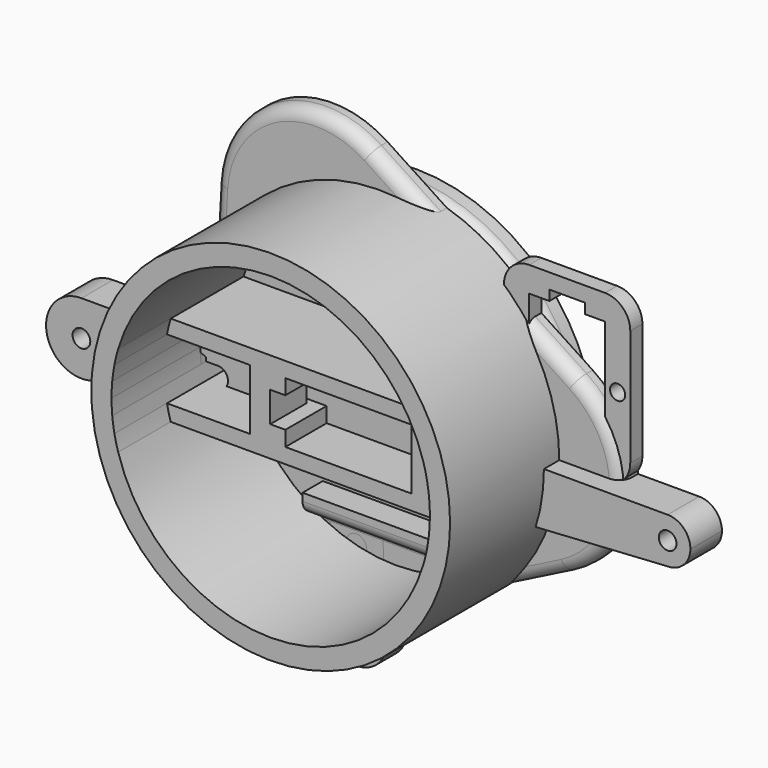
from build123d import *

# Parameters (mm, degrees)
F0_R          = 35.5
F0_W          = 29
F0_H          = 4
F0_R_2        = 1
F1_DEPTH      = 5
F2_DEPTH      = 5
F0_R_3        = 1.75
F3_DEPTH      = 3
F4_R          = 1.5
F5_DEPTH      = 3
F7_R          = 2.49999
F8_R          = 2.49999
F9_R          = 2.5
F11_DEPTH     = 31
F10_W         = 4
F10_H         = 3
F10_W_2       = 3
F12_DEPTH     = 18
F13_DEPTH     = 9
F14_DEPTH     = 9
F15_T4_DEPTH  = 14.302926823
F15_S5_R      = 31.5
F15_T6_DEPTH  = 9
F15_S7_R      = 35.5
F15_T8_DEPTH  = 9
F15_T12_DEPTH = 14.302926823
F15_S13_R     = 31.5
F15_T14_DEPTH = 9
F15_S15_R     = 35.5
F15_T16_DEPTH = 9
F17_DEPTH     = 4
F18_R         = 2.5
F6_R          = 2
F19_DEPTH     = 5
F20_DEPTH     = 3
F21_R         = 1.75
F22_DEPTH     = 7.8
F23_R         = 15
F24_DEPTH     = 2
F25_DEPTH     = 8


# Not quite as in the source:
# - a fillet or chamfer that OpenCascade refuses, or shapes differently, is made with other operations: its cross-section is extruded or revolved along the edge and cut away or added
# - a fillet or chamfer is up to 0.001 mm smaller than in the source, because OpenCascade refuses the exact size


with BuildPart() as f1:
    # F0 (on Front) → F1 (new body)
    with BuildSketch(Plane.XZ):
        Circle(F0_R)
        with Locations((0, -23.522429496)):
            Rectangle(F0_W, F0_H, mode=Mode.SUBTRACT)
        Polygon((-17.0606780064, 2.7416863016), (-13.6559690168, 3.1554426533), (-11.5952910104, 0.4137563518), (-12.9393219936, -2.7416863016), (-16.3440309832, -3.1554426533), (-18.4047089896, -0.4137563518), align=None, mode=Mode.SUBTRACT)
        Circle(F0_R_2, mode=Mode.SUBTRACT)
        Polygon((13.9117840481, 3.1093030377), (17.1486274427, 2.497074178), (18.2368433946, -0.6122288597), (16.0882159519, -3.1093030377), (12.8513725573, -2.497074178), (11.7631566054, 0.6122288597), align=None, mode=Mode.SUBTRACT)
        with Locations((0, 22.477570504)):
            Rectangle(F0_W, F0_H, mode=Mode.SUBTRACT)
        with Locations((0, 22.477570504)):
            Rectangle(F0_W, F0_H)
        with Locations((0, -23.522429496)):
            Rectangle(F0_W, F0_H)
    extrude(amount=-F1_DEPTH)

    # F0 (on Front) → F2 (join)
    with BuildSketch(Plane.XZ):
        with Locations((0, 22.477570504)):
            Rectangle(F0_W, F0_H)
        with Locations((0, -23.522429496)):
            Rectangle(F0_W, F0_H)
    extrude(amount=F2_DEPTH)

    # F0 (on Front) → F3 (join)
    with BuildSketch(Plane.XZ):
        Polygon((18.2368433946, -0.6122288597), (17.1486274427, 2.497074178), (13.9117840481, 3.1093030377), (11.7631566054, 0.6122288597), (12.8513725573, -2.497074178), (16.0882159519, -3.1093030377), align=None)
        with Locations((15, 0)):
            Circle(F0_R_3, mode=Mode.SUBTRACT)
        Polygon((-11.5952910104, 0.4137563518), (-13.6559690168, 3.1554426533), (-17.0606780064, 2.7416863016), (-18.4047089896, -0.4137563518), (-16.3440309832, -3.1554426533), (-12.9393219936, -2.7416863016), align=None)
        with Locations((-15, 0)):
            Circle(F0_R_3, mode=Mode.SUBTRACT)
    extrude(amount=-F3_DEPTH)

    # F7 (radius 2.5 in the source; OpenCascade refuses exactly that, so slightly less here)
    f7_edges = [f1.edges().sort_by_distance(p)[0] for p in [
        (0, -5, -25.522429),
        (0, 0, -25.522429),
    ]]
    fillet(f7_edges, radius=F7_R)

    # F8 (radius 2.5 in the source; OpenCascade refuses exactly that, so slightly less here)
    f8_edges = [f1.edges().sort_by_distance(p)[0] for p in [
        (0, -5, 24.477571),
        (0, 0, 24.477571),
    ]]
    fillet(f8_edges, radius=F8_R)

    # F9
    f9_edges = [f1.edges().sort_by_distance(p)[0] for p in [
        (-35.5, 0, 0),
    ]]
    fillet(f9_edges, radius=F9_R)


with BuildPart() as f5:
    # F4 (on Front) → F5 (new body)
    with BuildSketch(Plane.XZ):
        with BuildLine():
            Line((43.7464710474, 31.4150267243), (28.7464710474, 31.4150267243))
            ThreePointArc((28.7464710474, 31.4150267243), (25.2109371415, 29.9505606303), (23.7464710474, 26.4150267243))
            Line((23.7464710474, 26.4150267243), (23.7464710474, 3.4150267243))
            ThreePointArc((23.7464710474, 3.4150267243), (25.2109371415, -0.1205071816), (28.7464710474, -1.5849732757))
            Line((28.7464710474, -1.5849732757), (43.7464710474, -1.5849732757))
            ThreePointArc((43.7464710474, -1.5849732757), (47.2820049533, -0.1205071816), (48.7464710474, 3.4150267243))
            Line((48.7464710474, 3.4150267243), (48.7464710474, 26.4150267243))
            ThreePointArc((48.7464710474, 26.4150267243), (47.2820049533, 29.9505606303), (43.7464710474, 31.4150267243))
        make_face()
        with Locations((26.2464710474, 14.9150267243)):
            Circle(F4_R, mode=Mode.SUBTRACT)
        Polygon((28.7464710474, 3.4150267243), (28.7464710474, 26.4150267243), (32.7464710474, 26.4150267243), (32.7464710474, 28.4150267243), (39.7464710474, 28.4150267243), (39.7464710474, 26.4150267243), (43.7464710474, 26.4150267243), (43.7464710474, 3.4150267243), align=None, mode=Mode.SUBTRACT)
        with Locations((46.2464710474, 14.9150267243)):
            Circle(F4_R, mode=Mode.SUBTRACT)
    extrude(amount=F5_DEPTH)


with BuildPart() as f11:
    # F10 (on Front) → F11 (new body)
    with BuildSketch(Plane.XZ):
        with BuildLine():
            ThreePointArc((-31.5, 0), (-31.4641839985, 1.5017074653), (-31.3568174406, 3))
            Line((-31.3568174406, 3), (-35.3730123116, 3))
            ThreePointArc((-35.3730123116, 3), (-35.5, 0), (-35.3730123116, -3))
            Line((-35.3730123116, -3), (-31.3568174406, -3))
            ThreePointArc((-31.3568174406, -3), (-31.4641839985, -1.5017074653), (-31.5, 0))
        make_face()
        with BuildLine():
            ThreePointArc((30.9232921921, 6), (31.3554915769, 3.0138261353), (31.5, 0))
            ThreePointArc((31.5, 0), (31.3554915769, -3.0138261353), (30.9232921921, -6))
            ThreePointArc((30.9232921921, -6), (30.5919015125, -7.5090320181), (30.1869176962, -9))
            ThreePointArc((30.1869176962, -9), (0, -31.5), (-30.1869176962, -9))
            ThreePointArc((-30.1869176962, -9), (-30.5919015125, -7.5090320181), (-30.9232921921, -6))
            ThreePointArc((-30.9232921921, -6), (-31.1761609882, -4.5052176457), (-31.3568174406, -3))
            Line((-31.3568174406, -3), (-35.3730123116, -3))
            ThreePointArc((-35.3730123116, -3), (1.5013432213, -35.4682388699), (35.5, 0))
            ThreePointArc((35.5, 0), (1.5013432213, 35.4682388699), (-35.3730123116, 3))
            Line((-35.3730123116, 3), (-31.3568174406, 3))
            ThreePointArc((-31.3568174406, 3), (-31.1761609882, 4.5052176457), (-30.9232921921, 6))
            ThreePointArc((-30.9232921921, 6), (-30.5919015125, 7.5090320181), (-30.1869176962, 9))
            ThreePointArc((-30.1869176962, 9), (0, 31.5), (30.1869176962, 9))
            ThreePointArc((30.1869176962, 9), (30.5919015125, 7.5090320181), (30.9232921921, 6))
        make_face()
    extrude(amount=F11_DEPTH)

    # F10 (on Front) → F12 (join)
    with BuildSketch(Plane.XZ):
        with BuildLine():
            Line((22.5, 6), (30.9232921921, 6))
            ThreePointArc((30.9232921921, 6), (30.5919015125, 7.5090320181), (30.1869176962, 9))
            Line((30.1869176962, 9), (-30.1869176962, 9))
            ThreePointArc((-30.1869176962, 9), (-30.5919015125, 7.5090320181), (-30.9232921921, 6))
            Line((-30.9232921921, 6), (-14.5, 6))
            Line((-14.5, 6), (-10.5, 6))
            Line((-10.5, 6), (-7.5, 6))
            Line((-7.5, 6), (17.5, 6))
            Line((17.5, 6), (22.5, 6))
        make_face()
        with BuildLine():
            ThreePointArc((30.1869176962, -9), (30.5919015125, -7.5090320181), (30.9232921921, -6))
            Line((30.9232921921, -6), (22.5, -6))
            Line((22.5, -6), (17.5, -6))
            Line((17.5, -6), (-7.5, -6))
            Line((-7.5, -6), (-10.5, -6))
            Line((-10.5, -6), (-14.5, -6))
            Line((-14.5, -6), (-30.9232921921, -6))
            ThreePointArc((-30.9232921921, -6), (-30.5919015125, -7.5090320181), (-30.1869176962, -9))
            Line((-30.1869176962, -9), (30.1869176962, -9))
        make_face()
        Polygon((22.5, -6), (22.5, 0), (22.5, 6), (17.5, 6), (17.5, -6), align=None)
        Polygon((-10.5, 3), (-14.5, 3), (-14.5, 0), (-14.5, -3), (-10.5, -3), align=None)
        with Locations((-12.5, 4.5)):
            Rectangle(F10_W, F10_H)
        with Locations((-9, 4.5)):
            Rectangle(F10_W_2, F10_H)
        with Locations((-9, -4.5)):
            Rectangle(F10_W_2, F10_H)
        with Locations((-12.5, -4.5)):
            Rectangle(F10_W, F10_H)
    extrude(amount=F12_DEPTH)

    # F10 (on Front) → F13 (cut)
    with BuildSketch(Plane.XZ):
        Polygon((-10.5, 3), (-14.5, 3), (-14.5, 0), (-14.5, -3), (-10.5, -3), align=None)
    extrude(amount=F13_DEPTH, mode=Mode.SUBTRACT)

    # F10 (on Front) → F14 (cut)
    with BuildSketch(Plane.XZ):
        with BuildLine():
            ThreePointArc((-31.5, 0), (-31.4641839985, 1.5017074653), (-31.3568174406, 3))
            Line((-31.3568174406, 3), (-35.3730123116, 3))
            ThreePointArc((-35.3730123116, 3), (-35.5, 0), (-35.3730123116, -3))
            Line((-35.3730123116, -3), (-31.3568174406, -3))
            ThreePointArc((-31.3568174406, -3), (-31.4641839985, -1.5017074653), (-31.5, 0))
        make_face()
    extrude(amount=F14_DEPTH, mode=Mode.SUBTRACT)

    # F15: chamfer of 2 on 2 edges, made by hand


with BuildPart() as f15_tool2:
    # F15_s3 → F15_t4 (new body)
    with BuildSketch(Plane.YZ.offset(-26.2134514646)):
        Polygon((-9, 1), (-7, 3), (-9, 3), align=None)
    extrude(amount=-F15_T4_DEPTH)

    # F15_s5 → F15_t6 (cut, symmetric)
    with BuildSketch(Plane.XZ.offset(8)):
        Circle(F15_S5_R)
    extrude(amount=F15_T6_DEPTH, both=True, mode=Mode.SUBTRACT)

    # F15_s7 → F15_t8 (intersect, symmetric)
    with BuildSketch(Plane.XZ.offset(8)):
        Circle(F15_S7_R)
    extrude(amount=F15_T8_DEPTH, both=True, mode=Mode.INTERSECT)


with BuildPart() as f11_1:
    add(f11.part)

    # F15_t1: union F15_tool2
    add(f15_tool2.part)


with BuildPart() as f15_tool10:
    # F15_s11 → F15_t12 (new body)
    with BuildSketch(Plane.YZ.offset(-40.5163782876)):
        Polygon((-7, -3), (-9, -1), (-9, -3), align=None)
    extrude(amount=F15_T12_DEPTH)

    # F15_s13 → F15_t14 (cut, symmetric)
    with BuildSketch(Plane.XZ.offset(8)):
        Circle(F15_S13_R)
    extrude(amount=F15_T14_DEPTH, both=True, mode=Mode.SUBTRACT)

    # F15_s15 → F15_t16 (intersect, symmetric)
    with BuildSketch(Plane.XZ.offset(8)):
        Circle(F15_S15_R)
    extrude(amount=F15_T16_DEPTH, both=True, mode=Mode.INTERSECT)


with BuildPart() as f11_2:
    add(f11_1.part)

    # F15_t9: union F15_tool10
    add(f15_tool10.part)

    # F16 (on face) → F17 (join)
    with BuildSketch(Plane.XZ):
        with BuildLine():
            ThreePointArc((-33.3783015345, 12.0887959148), (-16.0094790364, 31.6851160797), (10.0699705918, 34.0418226933))
            Line((10.0699705918, 34.0418226933), (-1.6776871675, 41.7275132948))
            ThreePointArc((-1.6776871675, 41.7275132948), (-21.6466195422, 42.8418470936), (-32.5961271076, 26.1054112701))
            Line((-32.5961271076, 26.1054112701), (-33.3783015345, 12.0887959148))
        make_face()
        with BuildLine():
            Line((38.90601289, 15.1763685051), (27.1583551307, 22.8620591067))
            ThreePointArc((27.1583551307, 22.8620591067), (33.3494498241, 12.1681632316), (35.5, 0))
            ThreePointArc((35.5, 0), (32.6196756356, -14.0073823904), (24.4460979476, -25.7417616945))
            Line((24.4460979476, -25.7417616945), (36.9759301338, -19.4108369407))
            ThreePointArc((36.9759301338, -19.4108369407), (47.9254376992, -2.6744011172), (38.90601289, 15.1763685051))
        make_face()
        with BuildLine():
            Line((-6.3098857823, -41.2817797753), (6.2199464039, -34.9508550215))
            ThreePointArc((6.2199464039, -34.9508550215), (-19.4353759286, -29.7071735867), (-34.5160685394, -8.3000609988))
            Line((-34.5160685394, -8.3000609988), (-35.2982429663, -22.3166763541))
            ThreePointArc((-35.2982429663, -22.3166763541), (-26.278818157, -40.1674459764), (-6.3098857823, -41.2817797753))
        make_face()
    extrude(amount=F17_DEPTH)

    # F18
    f18_edges = [f11_2.edges().sort_by_distance(p)[0] for p in [
        (47.925438, -4, -2.674401),
        (-26.278818, -4, -40.167446),
        (-21.64662, -4, 42.841847),
        (-34.907156, -4, -15.308369),
        (-0.04497, -4, -38.116317),
        (30.711014, -4, -22.576299),
        (33.032184, -4, 19.019214),
        (4.196142, -4, 37.884668),
        (-32.987214, -4, 19.097104),
    ]]
    fillet(f18_edges, radius=F18_R)


with BuildPart() as f19:
    # F6 (on Front) → F19 (new body)
    with BuildSketch(Plane.XZ):
        with BuildLine():
            Line((-13.8065919992, -45.0317585825), (-13.8285924066, -45.5451014222))
            ThreePointArc((-13.8285924066, -45.5451014222), (-7.8285924066, -51.5451014222), (-1.8285924066, -45.5451014222))
            Line((-1.8285924066, -45.5451014222), (-1.850592814, -45.0317585825))
            ThreePointArc((-1.850592814, -45.0317585825), (-2.7682693631, -42.3212635392), (-4.8370166993, -40.3440943285))
            Line((-4.8370166993, -40.3440943285), (-4.346375486, -45.1927304275))
            ThreePointArc((-4.346375486, -45.1927304275), (-4.3330410036, -45.3686917032), (-4.3285924066, -45.5451014222))
            ThreePointArc((-4.3285924066, -45.5451014222), (-7.8285924066, -49.0451014222), (-11.3285924066, -45.5451014222))
            ThreePointArc((-11.3285924066, -45.5451014222), (-11.3112225723, -45.1968384056), (-11.2592854759, -44.8520321152))
            Line((-11.2592854759, -44.8520321152), (-10.807781171, -40.3369890668))
            ThreePointArc((-10.807781171, -40.3369890668), (-12.8850754746, -42.3152439976), (-13.8065919992, -45.0317585825))
        make_face()
        with BuildLine():
            Line((-12.3285924066, -10.5451014222), (-13.8065919992, -45.0317585825))
            ThreePointArc((-13.8065919992, -45.0317585825), (-12.8850754746, -42.3152439976), (-10.807781171, -40.3369890668))
            Line((-10.807781171, -40.3369890668), (-10.0952782738, -33.2119600947))
            ThreePointArc((-10.0952782738, -33.2119600947), (-11.2414756107, -31.3211350781), (-11.0255877564, -29.1205942327))
            Line((-11.0255877564, -29.1205942327), (-10.3881177664, -14.2462944639))
            ThreePointArc((-10.3881177664, -14.2462944639), (-11.8140575061, -12.634615227), (-12.3285924066, -10.5451014222))
        make_face()
        with BuildLine():
            ThreePointArc((-4.8370166993, -40.3440943285), (-2.7682693631, -42.3212635392), (-1.850592814, -45.0317585825))
            Line((-1.850592814, -45.0317585825), (-3.3285924066, -10.5451014222))
            ThreePointArc((-3.3285924066, -10.5451014222), (-3.8431273071, -12.634615227), (-5.2690670468, -14.2462944639))
            Line((-5.2690670468, -14.2462944639), (-4.6315970567, -29.1205942327))
            ThreePointArc((-4.6315970567, -29.1205942327), (-4.4051815545, -29.8169131651), (-4.3285924066, -30.5451014222))
            ThreePointArc((-4.3285924066, -30.5451014222), (-4.6510429476, -32.01247303), (-5.5589806554, -33.2094704842))
            Line((-5.5589806554, -33.2094704842), (-4.8370166993, -40.3440943285))
        make_face()
        with BuildLine():
            Line((-10.0952782738, -33.2119600947), (-10.807781171, -40.3369890668))
            ThreePointArc((-10.807781171, -40.3369890668), (-7.8214523594, -39.5451056705), (-4.8370166993, -40.3440943285))
            Line((-4.8370166993, -40.3440943285), (-5.5589806554, -33.2094704842))
            ThreePointArc((-5.5589806554, -33.2094704842), (-7.8266715372, -34.045100895), (-10.0952782738, -33.2119600947))
        make_face()
        with BuildLine():
            ThreePointArc((-4.8370166993, -40.3440943285), (-7.8214523594, -39.5451056705), (-10.807781171, -40.3369890668))
            Line((-10.807781171, -40.3369890668), (-11.2592854759, -44.8520321152))
            ThreePointArc((-11.2592854759, -44.8520321152), (-7.656306273, -42.0493443528), (-4.346375486, -45.1927304275))
            Line((-4.346375486, -45.1927304275), (-4.8370166993, -40.3440943285))
        make_face()
        with BuildLine():
            ThreePointArc((-3.3285924066, -10.5451014222), (-7.8285924066, -6.0451014222), (-12.3285924066, -10.5451014222))
            ThreePointArc((-12.3285924066, -10.5451014222), (-11.8140575061, -12.634615227), (-10.3881177664, -14.2462944639))
            ThreePointArc((-10.3881177664, -14.2462944639), (-7.8285924066, -15.0451014222), (-5.2690670468, -14.2462944639))
            ThreePointArc((-5.2690670468, -14.2462944639), (-3.8431273071, -12.634615227), (-3.3285924066, -10.5451014222))
        make_face()
        with Locations((-7.8285924066, -10.5451014222)):
            Circle(F6_R, mode=Mode.SUBTRACT)
        with BuildLine():
            ThreePointArc((-11.0255877564, -29.1205942327), (-11.2414756107, -31.3211350781), (-10.0952782738, -33.2119600947))
            Line((-10.0952782738, -33.2119600947), (-9.8285924066, -30.5451014222))
            ThreePointArc((-9.8285924066, -30.5451014222), (-7.8285924066, -28.5451014222), (-5.8285924066, -30.5451014222))
            Line((-5.8285924066, -30.5451014222), (-5.5589806554, -33.2094704842))
            ThreePointArc((-5.5589806554, -33.2094704842), (-4.6510429476, -32.01247303), (-4.3285924066, -30.5451014222))
            ThreePointArc((-4.3285924066, -30.5451014222), (-4.4051815545, -29.8169131651), (-4.6315970567, -29.1205942327))
            ThreePointArc((-4.6315970567, -29.1205942327), (-7.8285924066, -27.0451014222), (-11.0255877564, -29.1205942327))
        make_face()
        with BuildLine():
            Line((-9.8285924066, -30.5451014222), (-10.0952782738, -33.2119600947))
            ThreePointArc((-10.0952782738, -33.2119600947), (-7.8266715372, -34.045100895), (-5.5589806554, -33.2094704842))
            Line((-5.5589806554, -33.2094704842), (-5.8285924066, -30.5451014222))
            ThreePointArc((-5.8285924066, -30.5451014222), (-7.8285924066, -32.5451014222), (-9.8285924066, -30.5451014222))
        make_face()
        with BuildLine():
            ThreePointArc((-4.346375486, -45.1927304275), (-7.656306273, -42.0493443528), (-11.2592854759, -44.8520321152))
            Line((-11.2592854759, -44.8520321152), (-11.3285924066, -45.5451014222))
            ThreePointArc((-11.3285924066, -45.5451014222), (-7.8285924066, -49.0451014222), (-4.3285924066, -45.5451014222))
            ThreePointArc((-4.3285924066, -45.5451014222), (-4.3330410036, -45.3686917032), (-4.346375486, -45.1927304275))
        make_face()
        with Locations((-7.8285924066, -45.5451014222)):
            Circle(F6_R, mode=Mode.SUBTRACT)
        with BuildLine():
            ThreePointArc((-5.2690670468, -14.2462944639), (-7.8285924066, -15.0451014222), (-10.3881177664, -14.2462944639))
            Line((-10.3881177664, -14.2462944639), (-11.0255877564, -29.1205942327))
            ThreePointArc((-11.0255877564, -29.1205942327), (-7.8285924066, -27.0451014222), (-4.6315970567, -29.1205942327))
            Line((-4.6315970567, -29.1205942327), (-5.2690670468, -14.2462944639))
        make_face()
        with BuildLine():
            ThreePointArc((-5.8285924066, -30.5451014222), (-7.8285924066, -28.5451014222), (-9.8285924066, -30.5451014222))
            ThreePointArc((-9.8285924066, -30.5451014222), (-7.8285924066, -32.5451014222), (-5.8285924066, -30.5451014222))
        make_face()
    extrude(amount=-F19_DEPTH)

    # F6 (on Front) → F20 (cut)
    with BuildSketch(Plane.XZ):
        with BuildLine():
            Line((-10.0952782738, -33.2119600947), (-10.807781171, -40.3369890668))
            ThreePointArc((-10.807781171, -40.3369890668), (-7.8214523594, -39.5451056705), (-4.8370166993, -40.3440943285))
            Line((-4.8370166993, -40.3440943285), (-5.5589806554, -33.2094704842))
            ThreePointArc((-5.5589806554, -33.2094704842), (-7.8266715372, -34.045100895), (-10.0952782738, -33.2119600947))
        make_face()
        with BuildLine():
            ThreePointArc((-4.8370166993, -40.3440943285), (-7.8214523594, -39.5451056705), (-10.807781171, -40.3369890668))
            Line((-10.807781171, -40.3369890668), (-11.2592854759, -44.8520321152))
            ThreePointArc((-11.2592854759, -44.8520321152), (-7.656306273, -42.0493443528), (-4.346375486, -45.1927304275))
            Line((-4.346375486, -45.1927304275), (-4.8370166993, -40.3440943285))
        make_face()
        with BuildLine():
            ThreePointArc((-4.346375486, -45.1927304275), (-7.656306273, -42.0493443528), (-11.2592854759, -44.8520321152))
            Line((-11.2592854759, -44.8520321152), (-11.3285924066, -45.5451014222))
            ThreePointArc((-11.3285924066, -45.5451014222), (-7.8285924066, -49.0451014222), (-4.3285924066, -45.5451014222))
            ThreePointArc((-4.3285924066, -45.5451014222), (-4.3330410036, -45.3686917032), (-4.346375486, -45.1927304275))
        make_face()
        with Locations((-7.8285924066, -45.5451014222)):
            Circle(F6_R, mode=Mode.SUBTRACT)
        with BuildLine():
            Line((-9.8285924066, -30.5451014222), (-10.0952782738, -33.2119600947))
            ThreePointArc((-10.0952782738, -33.2119600947), (-7.8266715372, -34.045100895), (-5.5589806554, -33.2094704842))
            Line((-5.5589806554, -33.2094704842), (-5.8285924066, -30.5451014222))
            ThreePointArc((-5.8285924066, -30.5451014222), (-7.8285924066, -32.5451014222), (-9.8285924066, -30.5451014222))
        make_face()
        with BuildLine():
            ThreePointArc((-5.8285924066, -30.5451014222), (-7.8285924066, -28.5451014222), (-9.8285924066, -30.5451014222))
            ThreePointArc((-9.8285924066, -30.5451014222), (-7.8285924066, -32.5451014222), (-5.8285924066, -30.5451014222))
        make_face()
    extrude(amount=-F20_DEPTH, mode=Mode.SUBTRACT)


with BuildPart() as f22:
    # F21 (on Front) → F22 (new body)
    with BuildSketch(Plane.XZ):
        with BuildLine():
            Line((59.9833536744, 0), (-56.0166463256, 0))
            ThreePointArc((-56.0166463256, 0), (-52.2996435239, -1.0683990212), (-49.7172813379, -3.9474599509))
            ThreePointArc((-49.7172813379, -3.9474599509), (-48.9900218702, -3.2528480177), (-48.0166463256, -3))
            Line((-48.0166463256, -3), (-29.0166463256, -3))
            ThreePointArc((-29.0166463256, -3), (-28.0341015748, -3.2579879987), (-27.3050415779, -3.9653941874))
            ThreePointArc((-27.3050415779, -3.9653941874), (-19.4385197238, -0.2198002349), (-14.0162597141, -7.039678278))
            ThreePointArc((-14.0162597141, -7.039678278), (-15.7686933898, -11.6725011402), (-20.1485590491, -13.9856912031))
            Line((-20.1485590491, -13.9856912031), (59.9833536744, -9))
            ThreePointArc((59.9833536744, -9), (55.4833536744, -4.5), (59.9833536744, 0))
        make_face()
        with BuildLine():
            ThreePointArc((-49.0166463256, -7), (-49.2551655416, -8.8117333157), (-49.9544684991, -10.5))
            Line((-49.9544684991, -10.5), (-27.1011733191, -10.5))
            ThreePointArc((-27.1011733191, -10.5), (-27.8218206103, -8.6780741057), (-28.0093082494, -6.7277933905))
            ThreePointArc((-28.0093082494, -6.7277933905), (-28.494912093, -6.9307494375), (-29.0166463256, -7))
            Line((-29.0166463256, -7), (-48.0166463256, -7))
            ThreePointArc((-48.0166463256, -7), (-48.537212712, -6.9310646383), (-49.0218936662, -6.7290106374))
            ThreePointArc((-49.0218936662, -6.7290106374), (-49.0179582837, -6.8644799192), (-49.0166463256, -7))
        make_face()
        with BuildLine():
            ThreePointArc((-49.7172813379, -3.9474599509), (-52.2996435239, -1.0683990212), (-56.0166463256, 0))
            ThreePointArc((-56.0166463256, 0), (-62.0788241521, -10.5), (-49.9544684991, -10.5))
            ThreePointArc((-49.9544684991, -10.5), (-49.2551655416, -8.8117333157), (-49.0166463256, -7))
            ThreePointArc((-49.0166463256, -7), (-49.0179582837, -6.8644799192), (-49.0218936662, -6.7290106374))
            ThreePointArc((-49.0218936662, -6.7290106374), (-49.9569313259, -5.4850712501), (-49.7172813379, -3.9474599509))
        make_face()
        with Locations((-56.0166463256, -7)):
            Circle(F21_R, mode=Mode.SUBTRACT)
        with BuildLine():
            Line((-29.0166463256, -3), (-48.0166463256, -3))
            ThreePointArc((-48.0166463256, -3), (-46.6024327632, -3.5857864376), (-46.0166463256, -5))
            ThreePointArc((-46.0166463256, -5), (-46.6024327632, -6.4142135624), (-48.0166463256, -7))
            Line((-48.0166463256, -7), (-29.0166463256, -7))
            ThreePointArc((-29.0166463256, -7), (-31.0166463256, -5), (-29.0166463256, -3))
        make_face()
        with BuildLine():
            ThreePointArc((-29.0166463256, -7), (-28.494912093, -6.9307494375), (-28.0093082494, -6.7277933905))
            ThreePointArc((-28.0093082494, -6.7277933905), (-27.7992875798, -5.3103625251), (-27.3050415779, -3.9653941874))
            ThreePointArc((-27.3050415779, -3.9653941874), (-28.0341015748, -3.2579879987), (-29.0166463256, -3))
            ThreePointArc((-29.0166463256, -3), (-31.0166463256, -5), (-29.0166463256, -7))
        make_face()
        with BuildLine():
            ThreePointArc((-48.0166463256, -3), (-48.9900218702, -3.2528480177), (-49.7172813379, -3.9474599509))
            ThreePointArc((-49.7172813379, -3.9474599509), (-49.2256488246, -5.3022506247), (-49.0218936662, -6.7290106374))
            ThreePointArc((-49.0218936662, -6.7290106374), (-48.537212712, -6.9310646383), (-48.0166463256, -7))
            ThreePointArc((-48.0166463256, -7), (-46.6024327632, -6.4142135624), (-46.0166463256, -5))
            ThreePointArc((-46.0166463256, -5), (-46.6024327632, -3.5857864376), (-48.0166463256, -3))
        make_face()
        with BuildLine():
            ThreePointArc((-49.0218936662, -6.7290106374), (-49.2256488246, -5.3022506247), (-49.7172813379, -3.9474599509))
            ThreePointArc((-49.7172813379, -3.9474599509), (-49.9569313259, -5.4850712501), (-49.0218936662, -6.7290106374))
        make_face()
        with BuildLine():
            ThreePointArc((-28.0093082494, -6.7277933905), (-27.8218206103, -8.6780741057), (-27.1011733191, -10.5))
            ThreePointArc((-27.1011733191, -10.5), (-24.5360429422, -13.0903911308), (-21.0162597141, -14.039678278))
            Line((-21.0162597141, -14.039678278), (-20.1485590491, -13.9856912031))
            ThreePointArc((-20.1485590491, -13.9856912031), (-15.7686933898, -11.6725011402), (-14.0162597141, -7.039678278))
            ThreePointArc((-14.0162597141, -7.039678278), (-19.4385197238, -0.2198002349), (-27.3050415779, -3.9653941874))
            ThreePointArc((-27.3050415779, -3.9653941874), (-27.0900937704, -4.4629755571), (-27.0166463256, -5))
            ThreePointArc((-27.0166463256, -5), (-27.2824784917, -5.9963242062), (-28.0093082494, -6.7277933905))
        make_face()
        with Locations((-21.0162597141, -7.039678278)):
            Circle(F21_R, mode=Mode.SUBTRACT)
        with BuildLine():
            ThreePointArc((-27.3050415779, -3.9653941874), (-27.7992875798, -5.3103625251), (-28.0093082494, -6.7277933905))
            ThreePointArc((-28.0093082494, -6.7277933905), (-27.2824784917, -5.9963242062), (-27.0166463256, -5))
            ThreePointArc((-27.0166463256, -5), (-27.0900937704, -4.4629755571), (-27.3050415779, -3.9653941874))
        make_face()
        with BuildLine():
            ThreePointArc((64.4833536744, -4.5), (63.1653341898, -1.3180194847), (59.9833536744, 0))
            ThreePointArc((59.9833536744, 0), (55.4833536744, -4.5), (59.9833536744, -9))
            ThreePointArc((59.9833536744, -9), (63.1653341898, -7.6819805153), (64.4833536744, -4.5))
        make_face()
        with Locations((59.9833540618, -4.5)):
            Circle(F21_R, mode=Mode.SUBTRACT)
    extrude(amount=F22_DEPTH)

    # F23
    f23_edges = [f22.edges().sort_by_distance(p)[0] for p in [
        (-49.954468, -3.9, -10.5),
        (-27.101173, -3.9, -10.5),
    ]]
    fillet(f23_edges, radius=F23_R)

    # F21 (on Front) → F24 (cut)
    with BuildSketch(Plane.XZ):
        with BuildLine():
            ThreePointArc((-29.0166463256, -7), (-28.494912093, -6.9307494375), (-28.0093082494, -6.7277933905))
            ThreePointArc((-28.0093082494, -6.7277933905), (-27.7992875798, -5.3103625251), (-27.3050415779, -3.9653941874))
            ThreePointArc((-27.3050415779, -3.9653941874), (-28.0341015748, -3.2579879987), (-29.0166463256, -3))
            ThreePointArc((-29.0166463256, -3), (-31.0166463256, -5), (-29.0166463256, -7))
        make_face()
        with BuildLine():
            Line((-29.0166463256, -3), (-48.0166463256, -3))
            ThreePointArc((-48.0166463256, -3), (-46.6024327632, -3.5857864376), (-46.0166463256, -5))
            ThreePointArc((-46.0166463256, -5), (-46.6024327632, -6.4142135624), (-48.0166463256, -7))
            Line((-48.0166463256, -7), (-29.0166463256, -7))
            ThreePointArc((-29.0166463256, -7), (-31.0166463256, -5), (-29.0166463256, -3))
        make_face()
        with BuildLine():
            ThreePointArc((-48.0166463256, -3), (-48.9900218702, -3.2528480177), (-49.7172813379, -3.9474599509))
            ThreePointArc((-49.7172813379, -3.9474599509), (-49.2256488246, -5.3022506247), (-49.0218936662, -6.7290106374))
            ThreePointArc((-49.0218936662, -6.7290106374), (-48.537212712, -6.9310646383), (-48.0166463256, -7))
            ThreePointArc((-48.0166463256, -7), (-46.6024327632, -6.4142135624), (-46.0166463256, -5))
            ThreePointArc((-46.0166463256, -5), (-46.6024327632, -3.5857864376), (-48.0166463256, -3))
        make_face()
        with BuildLine():
            ThreePointArc((-27.3050415779, -3.9653941874), (-27.7992875798, -5.3103625251), (-28.0093082494, -6.7277933905))
            ThreePointArc((-28.0093082494, -6.7277933905), (-27.2824784917, -5.9963242062), (-27.0166463256, -5))
            ThreePointArc((-27.0166463256, -5), (-27.0900937704, -4.4629755571), (-27.3050415779, -3.9653941874))
        make_face()
        with BuildLine():
            ThreePointArc((-49.0218936662, -6.7290106374), (-49.2256488246, -5.3022506247), (-49.7172813379, -3.9474599509))
            ThreePointArc((-49.7172813379, -3.9474599509), (-49.9569313259, -5.4850712501), (-49.0218936662, -6.7290106374))
        make_face()
    extrude(amount=F24_DEPTH, mode=Mode.SUBTRACT)

    # F21 (on Front) → F25 (cut)
    with BuildSketch(Plane.XZ):
        with BuildLine():
            Line((-29.0166463256, -3), (-48.0166463256, -3))
            ThreePointArc((-48.0166463256, -3), (-46.6024327632, -3.5857864376), (-46.0166463256, -5))
            ThreePointArc((-46.0166463256, -5), (-46.6024327632, -6.4142135624), (-48.0166463256, -7))
            Line((-48.0166463256, -7), (-29.0166463256, -7))
            ThreePointArc((-29.0166463256, -7), (-31.0166463256, -5), (-29.0166463256, -3))
        make_face()
        with BuildLine():
            ThreePointArc((-48.0166463256, -3), (-48.9900218702, -3.2528480177), (-49.7172813379, -3.9474599509))
            ThreePointArc((-49.7172813379, -3.9474599509), (-49.2256488246, -5.3022506247), (-49.0218936662, -6.7290106374))
            ThreePointArc((-49.0218936662, -6.7290106374), (-48.537212712, -6.9310646383), (-48.0166463256, -7))
            ThreePointArc((-48.0166463256, -7), (-46.6024327632, -6.4142135624), (-46.0166463256, -5))
            ThreePointArc((-46.0166463256, -5), (-46.6024327632, -3.5857864376), (-48.0166463256, -3))
        make_face()
        with BuildLine():
            ThreePointArc((-49.0218936662, -6.7290106374), (-49.2256488246, -5.3022506247), (-49.7172813379, -3.9474599509))
            ThreePointArc((-49.7172813379, -3.9474599509), (-49.9569313259, -5.4850712501), (-49.0218936662, -6.7290106374))
        make_face()
        with BuildLine():
            ThreePointArc((-29.0166463256, -7), (-28.494912093, -6.9307494375), (-28.0093082494, -6.7277933905))
            ThreePointArc((-28.0093082494, -6.7277933905), (-27.7992875798, -5.3103625251), (-27.3050415779, -3.9653941874))
            ThreePointArc((-27.3050415779, -3.9653941874), (-28.0341015748, -3.2579879987), (-29.0166463256, -3))
            ThreePointArc((-29.0166463256, -3), (-31.0166463256, -5), (-29.0166463256, -7))
        make_face()
        with BuildLine():
            ThreePointArc((-27.3050415779, -3.9653941874), (-27.7992875798, -5.3103625251), (-28.0093082494, -6.7277933905))
            ThreePointArc((-28.0093082494, -6.7277933905), (-27.2824784917, -5.9963242062), (-27.0166463256, -5))
            ThreePointArc((-27.0166463256, -5), (-27.0900937704, -4.4629755571), (-27.3050415779, -3.9653941874))
        make_face()
    extrude(amount=F25_DEPTH, mode=Mode.SUBTRACT)


solid = Compound([f1.part, f5.part, f11_2.part, f19.part, f22.part])
